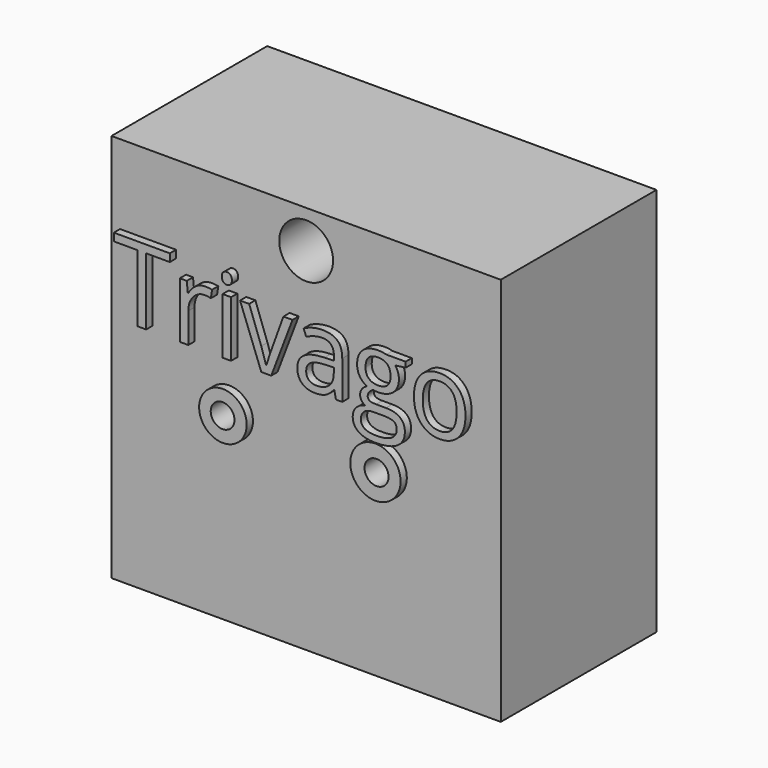
from build123d import *

# Parameters (mm, degrees)
F0_W          = 50
F0_H          = 50
F1_DEPTH      = 25
F2_R          = 3.4599369672
F3_DEPTH      = 25
F4_R          = 1.5264639974
F5_DEPTH      = 25
F4_R_2        = 1.5431370668
F6_DEPTH      = 25
F7_R          = 3.0555852486
F7_R_2        = 1.5264639974
F8_DEPTH      = 1
F9_R          = 3.2336533746
F9_R_2        = 1.5431370668
F10_DEPTH     = 1
F12_TEXT_SIZE = 13.4494401411
F13_DEPTH     = 1


# Not quite as in the source:
# - Text() gives the source's letters only with a copy of the font that has no kerning and outlines rounded to 1/6400 em; it was checked with that copy


with BuildPart() as f1:
    # F0 (on Front) → F1 (new body)
    with BuildSketch(Plane.XZ):
        Rectangle(F0_W, F0_H)
    extrude(amount=F1_DEPTH)

    # F2 (on face) → F3 (cut, through all)
    with BuildSketch(Plane.XZ.offset(25)):
        with Locations((0, 20.151603967)):
            Circle(F2_R)
    extrude(amount=-F3_DEPTH, mode=Mode.SUBTRACT)

    # F4 (on face) → F5 (cut, through all)
    with BuildSketch(Plane.XZ.offset(25)):
        with Locations((-9.9316518754, -1.3187045697)):
            Circle(F4_R)
    extrude(amount=-F5_DEPTH, mode=Mode.SUBTRACT)

    # F4 (on face) → F6 (cut, through all)
    with BuildSketch(Plane.XZ.offset(25)):
        with Locations((9.8427543417, -1.3187045697)):
            Circle(F4_R_2)
    extrude(amount=-F6_DEPTH, mode=Mode.SUBTRACT)

    # F7 (on face) → F8 (join)
    with BuildSketch(Plane.XZ.offset(25)):
        with Locations((-9.8922569305, -1.3422907796)):
            Circle(F7_R)
        with Locations((-9.9316518754, -1.3187045697)):
            Circle(F7_R_2, mode=Mode.SUBTRACT)
    extrude(amount=F8_DEPTH)

    # F9 (on face) → F10 (join)
    with BuildSketch(Plane.XZ.offset(25)):
        with Locations((9.699575603, -1.3277598191)):
            Circle(F9_R)
        with Locations((9.8427543417, -1.3187045697)):
            Circle(F9_R_2, mode=Mode.SUBTRACT)
    extrude(amount=F10_DEPTH)

    # F12 (on face) → F13 (join)
    with BuildSketch(Plane.XZ.offset(25)):
        with Locations((-24.0253265947, 5.2297543734)):
            Text('Trivago', F12_TEXT_SIZE, font='Open Sans', text_align=(TextAlign.LEFT, TextAlign.BOTTOM))
    extrude(amount=F13_DEPTH)


solid = f1.part
